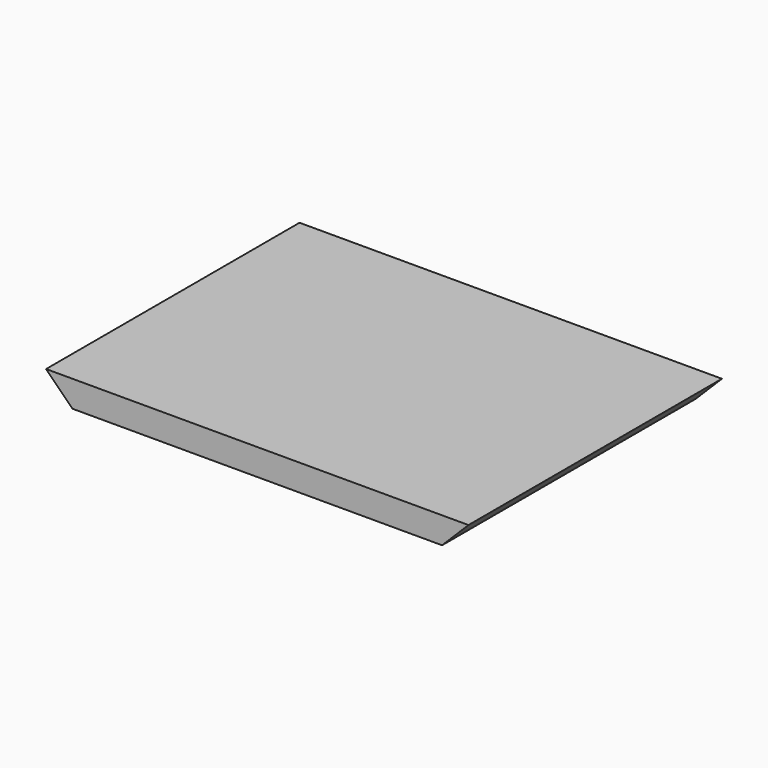
from build123d import *

# Parameters (mm, degrees)
F0_W     = 400
F0_H     = 300
F1_DEPTH = 25
F2_SIZE  = 24.99999


# Not quite as in the source:
# - a fillet or chamfer is up to 0.001 mm smaller than in the source, because OpenCascade refuses the exact size


with BuildPart() as f1:
    # F0 (on Top) → F1 (new body)
    with BuildSketch(Plane.XY):
        Rectangle(F0_W, F0_H)
    extrude(amount=-F1_DEPTH)

    # F2 (size 25 in the source; OpenCascade refuses exactly that, so slightly less here)
    f2_edges = [f1.edges().sort_by_distance(p)[0] for p in [
        (-200, 0, -25),
        (200, 0, -25),
    ]]
    chamfer(f2_edges, length=F2_SIZE)


solid = f1.part
